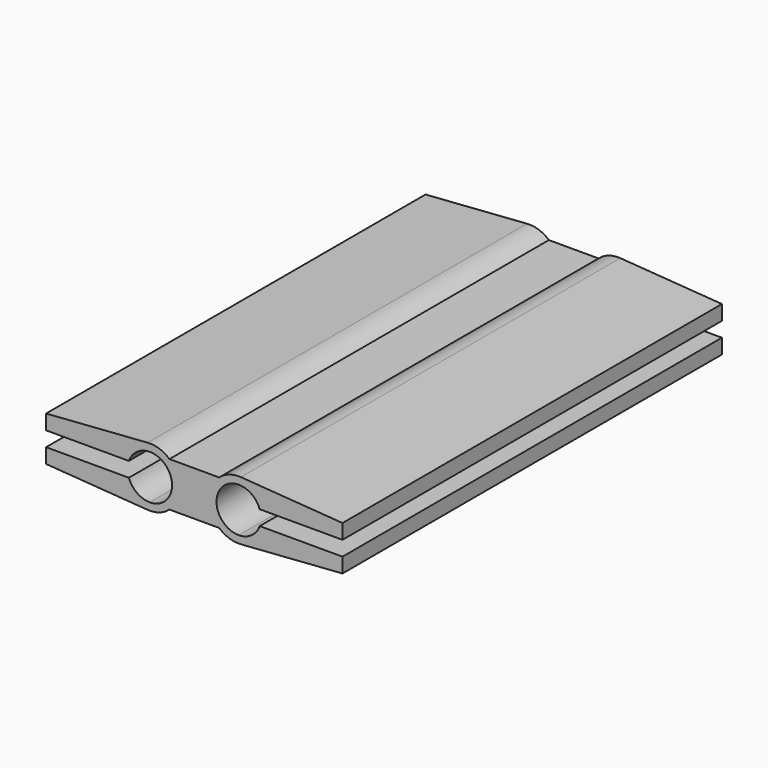
from build123d import *

# Parameters (mm, degrees)
F1_DEPTH = 32


# Not quite as in the source:
# - a feature names something its author has since deleted; it is built from what else it names


with BuildPart() as f1:
    # F0 (on Front) → F1 (new body)
    with BuildSketch(Plane.XZ):
        with BuildLine():
            Line((0.200491711, 11.3311297744), (-6.6555393256, 10.8363182701))
            Line((-6.6555393256, 10.8363182701), (-0.9784149812, 10.8363182701))
            ThreePointArc((-0.9784149812, 10.8363182701), (-0.429566386, 11.1804663417), (0.200491711, 11.3311297744))
        make_face()
        with BuildLine():
            Line((-0.9784149812, 10.8363182701), (-6.6555393256, 10.8363182701))
            Line((-6.6555393256, 10.8363182701), (-6.6555393256, 9.8363182701))
            Line((-6.6555393256, 9.8363182701), (-1.5920309988, 9.8363182701))
            ThreePointArc((-1.5920309988, 9.8363182701), (-1.3602002438, 10.382325514), (-0.9784149812, 10.8363182701))
        make_face()
        with BuildLine():
            ThreePointArc((0.200491711, 11.3311297744), (-0.429566386, 11.1804663417), (-0.9784149812, 10.8363182701))
            Line((-0.9784149812, 10.8363182701), (0.3444606744, 10.8363182701))
            Line((0.3444606744, 10.8363182701), (1.6673363299, 10.8363182701))
            ThreePointArc((1.6673363299, 10.8363182701), (0.9837296736, 11.2314001012), (0.200491711, 11.3311297744))
        make_face()
        with BuildLine():
            Line((0.3444606744, 10.8363182701), (-0.9784149812, 10.8363182701))
            ThreePointArc((-0.9784149812, 10.8363182701), (-1.3602002438, 10.382325514), (-1.5920309988, 9.8363182701))
            Line((-1.5920309988, 9.8363182701), (-1.069752888, 9.8363182701))
            ThreePointArc((-1.069752888, 9.8363182701), (-0.5215647294, 10.5610631415), (0.3444606744, 10.8363182701))
        make_face()
        with BuildLine():
            Line((1.6673363299, 10.8363182701), (0.3444606744, 10.8363182701))
            ThreePointArc((0.3444606744, 10.8363182701), (1.4051208461, 10.3969784419), (1.8444606744, 9.3363182701))
            ThreePointArc((1.8444606744, 9.3363182701), (1.4051208461, 8.2756580983), (0.3444606744, 7.8363182701))
            Line((0.3444606744, 7.8363182701), (1.6673363299, 7.8363182701))
            ThreePointArc((1.6673363299, 7.8363182701), (2.1673363299, 8.5134426146), (2.3444606744, 9.3363182701))
            ThreePointArc((2.3444606744, 9.3363182701), (2.1673363299, 10.1591939256), (1.6673363299, 10.8363182701))
        make_face()
        with BuildLine():
            Line((-1.5920309988, 8.8363182701), (-6.6555393256, 8.8363182701))
            Line((-6.6555393256, 8.8363182701), (-6.6555393256, 7.8363182701))
            Line((-6.6555393256, 7.8363182701), (-0.9784149812, 7.8363182701))
            ThreePointArc((-0.9784149812, 7.8363182701), (-1.3602002438, 8.2903110262), (-1.5920309988, 8.8363182701))
        make_face()
        with BuildLine():
            Line((5.0215850188, 10.8363182701), (1.6673363299, 10.8363182701))
            ThreePointArc((1.6673363299, 10.8363182701), (2.1673363299, 10.1591939256), (2.3444606744, 9.3363182701))
            ThreePointArc((2.3444606744, 9.3363182701), (2.1673363299, 8.5134426146), (1.6673363299, 7.8363182701))
            Line((1.6673363299, 7.8363182701), (5.0215850188, 7.8363182701))
            ThreePointArc((5.0215850188, 7.8363182701), (4.3444606744, 9.3363182701), (5.0215850188, 10.8363182701))
        make_face()
        with BuildLine():
            Line((-1.069752888, 8.8363182701), (-1.5920309988, 8.8363182701))
            ThreePointArc((-1.5920309988, 8.8363182701), (-1.3602002438, 8.2903110262), (-0.9784149812, 7.8363182701))
            Line((-0.9784149812, 7.8363182701), (0.3444606744, 7.8363182701))
            ThreePointArc((0.3444606744, 7.8363182701), (-0.5215647294, 8.1115733987), (-1.069752888, 8.8363182701))
        make_face()
        with BuildLine():
            Line((-0.9784149812, 7.8363182701), (-6.6555393256, 7.8363182701))
            Line((-6.6555393256, 7.8363182701), (0.200491711, 7.3415067658))
            ThreePointArc((0.200491711, 7.3415067658), (-0.429566386, 7.4921701986), (-0.9784149812, 7.8363182701))
        make_face()
        with BuildLine():
            ThreePointArc((6.4884296377, 11.3311297744), (5.7051916751, 11.2314001012), (5.0215850188, 10.8363182701))
            Line((5.0215850188, 10.8363182701), (6.344460699, 10.8363182701))
            Line((6.344460699, 10.8363182701), (7.6673363299, 10.8363182701))
            ThreePointArc((7.6673363299, 10.8363182701), (7.1184877347, 11.1804663417), (6.4884296377, 11.3311297744))
        make_face()
        with BuildLine():
            Line((6.344460699, 10.8363182701), (5.0215850188, 10.8363182701))
            ThreePointArc((5.0215850188, 10.8363182701), (4.3444606744, 9.3363182701), (5.0215850188, 7.8363182701))
            Line((5.0215850188, 7.8363182701), (6.3444606473, 7.8363182701))
            ThreePointArc((6.3444606473, 7.8363182701), (4.8444606744, 9.336318296), (6.344460699, 10.8363182701))
        make_face()
        with BuildLine():
            Line((1.6673363299, 7.8363182701), (0.3444606744, 7.8363182701))
            Line((0.3444606744, 7.8363182701), (-0.9784149812, 7.8363182701))
            ThreePointArc((-0.9784149812, 7.8363182701), (-0.429566386, 7.4921701986), (0.200491711, 7.3415067658))
            ThreePointArc((0.200491711, 7.3415067658), (0.9837296736, 7.441236439), (1.6673363299, 7.8363182701))
        make_face()
        with BuildLine():
            Line((7.6673363299, 10.8363182701), (6.344460699, 10.8363182701))
            ThreePointArc((6.344460699, 10.8363182701), (7.2104860882, 10.5610631344), (7.7586742367, 9.8363182701))
            Line((7.7586742367, 9.8363182701), (8.2809523475, 9.8363182701))
            ThreePointArc((8.2809523475, 9.8363182701), (8.0491215925, 10.382325514), (7.6673363299, 10.8363182701))
        make_face()
        with BuildLine():
            Line((13.3444606744, 10.8363182701), (6.4884296377, 11.3311297744))
            ThreePointArc((6.4884296377, 11.3311297744), (7.1184877347, 11.1804663417), (7.6673363299, 10.8363182701))
            Line((7.6673363299, 10.8363182701), (13.3444606744, 10.8363182701))
        make_face()
        with BuildLine():
            Line((6.3444606473, 7.8363182701), (5.0215850188, 7.8363182701))
            ThreePointArc((5.0215850188, 7.8363182701), (5.7051916751, 7.441236439), (6.4884296377, 7.3415067658))
            ThreePointArc((6.4884296377, 7.3415067658), (7.1184877347, 7.4921701986), (7.6673363299, 7.8363182701))
            Line((7.6673363299, 7.8363182701), (6.3444606473, 7.8363182701))
        make_face()
        with BuildLine():
            Line((13.3444606744, 10.8363182701), (7.6673363299, 10.8363182701))
            ThreePointArc((7.6673363299, 10.8363182701), (8.0491215925, 10.382325514), (8.2809523475, 9.8363182701))
            Line((8.2809523475, 9.8363182701), (13.3444606744, 9.8363182701))
            Line((13.3444606744, 9.8363182701), (13.3444606744, 10.8363182701))
        make_face()
        with BuildLine():
            ThreePointArc((7.7586742367, 8.8363182701), (7.2104860671, 8.1115733909), (6.3444606473, 7.8363182701))
            Line((6.3444606473, 7.8363182701), (7.6673363299, 7.8363182701))
            ThreePointArc((7.6673363299, 7.8363182701), (8.0491215925, 8.2903110262), (8.2809523475, 8.8363182701))
            Line((8.2809523475, 8.8363182701), (7.7586742367, 8.8363182701))
        make_face()
        with BuildLine():
            ThreePointArc((7.6673363299, 7.8363182701), (7.1184877347, 7.4921701986), (6.4884296377, 7.3415067658))
            Line((6.4884296377, 7.3415067658), (13.3444606744, 7.8363182701))
            Line((13.3444606744, 7.8363182701), (7.6673363299, 7.8363182701))
        make_face()
        with BuildLine():
            ThreePointArc((8.2809523475, 8.8363182701), (8.0491215925, 8.2903110262), (7.6673363299, 7.8363182701))
            Line((7.6673363299, 7.8363182701), (13.3444606744, 7.8363182701))
            Line((13.3444606744, 7.8363182701), (13.3444606744, 8.8363182701))
            Line((13.3444606744, 8.8363182701), (8.2809523475, 8.8363182701))
        make_face()
    extrude(amount=F1_DEPTH)


solid = f1.part
